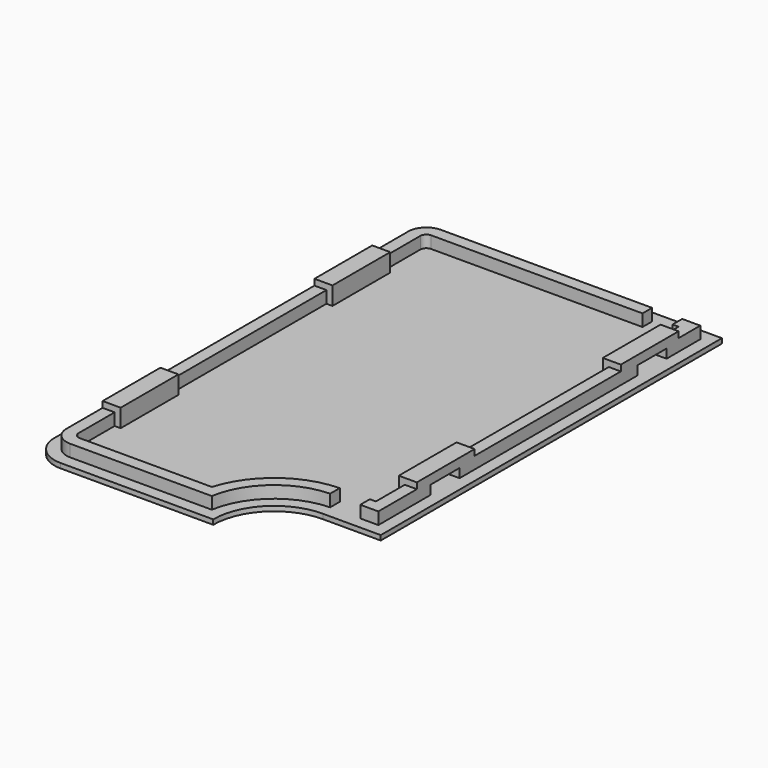
from build123d import *

# Parameters (mm, degrees)
F1_DEPTH  = 0.8
F2_R      = 5
F3_R      = 5
F5_DEPTH  = 3
F8_W      = 6
F8_H      = 1.5
F9_DEPTH  = 2
F11_DEPTH = 1.5
F12_DEPTH = 1.5
F6_W      = 6
F6_H      = 1.5
F13_DEPTH = 1
F14_W     = 2
F14_H     = 32
F14_H_2   = 30.375
F15_DEPTH = 2


# Not quite as in the source:
# - an extrude ends at something that could not be found from the text; its depth is read off the source's solid


with BuildPart() as f1:
    # F0 (on Top) → F1 (new body)
    with BuildSketch(Plane.XY):
        with BuildLine():
            Line((20.9010709455, 49.8366734011), (-29.2176790545, 49.8366734011))
            Line((-29.2176790545, 49.8366734011), (-29.2176790545, -31.1633265989))
            Line((-29.2176790545, -31.1633265989), (1.1573209455, -31.1633265989))
            ThreePointArc((1.1573209455, -31.1633265989), (4.122864786, -24.0038704394), (11.2823209455, -21.0383265989))
            Line((11.2823209455, -21.0383265989), (20.9010709455, -21.0383265989))
            Line((20.9010709455, -21.0383265989), (20.9010709455, 49.8366734011))
        make_face()
    extrude(amount=F1_DEPTH)

    # F2
    f2_edges = [f1.edges().sort_by_distance(p)[0] for p in [
        (-29.217679, 49.836673, 0.4),
    ]]
    fillet(f2_edges, radius=F2_R)

    # F3
    f3_edges = [f1.edges().sort_by_distance(p)[0] for p in [
        (-29.217679, -31.163327, 0.4),
    ]]
    fillet(f3_edges, radius=F3_R)

    # F4 (on face) → F5 (join)
    with BuildSketch(Plane.XY.offset(0.8)):
        with BuildLine():
            ThreePointArc((-24.2176790545, 47.8366734011), (-26.338999398, 46.9579937447), (-27.2176790545, 44.8366734011))
            Line((-27.2176790545, 44.8366734011), (-27.2176790545, -26.1633265989))
            ThreePointArc((-27.2176790545, -26.1633265989), (-26.338999398, -28.2846469425), (-24.2176790545, -29.1633265989))
            Line((-24.2176790545, -29.1633265989), (-0.6765930938, -29.1633265989))
            ThreePointArc((-0.6765930938, -29.1633265989), (3.4476025396, -21.9095267037), (11.2823209455, -19.0383265989))
            Line((11.2823209455, -19.0383265989), (18.9010709455, -19.0383265989))
            Line((18.9010709455, -19.0383265989), (18.9010709455, 47.8366734011))
            Line((18.9010709455, 47.8366734011), (-24.2176790545, 47.8366734011))
        make_face()
    extrude(amount=F5_DEPTH)

    # F8 (on face) → F9 (cut)
    with BuildSketch(Plane.YZ.offset(18.9010709455)):
        with Locations((-5.1633265989, 1.55)):
            Rectangle(F8_W, F8_H)
        with Locations((37.8366734011, 1.55)):
            Rectangle(F8_W, F8_H)
    extrude(amount=-F9_DEPTH, mode=Mode.SUBTRACT)

    # F10 (on face) → F11 (cut)
    with BuildSketch(Plane.XY.offset(3.8)):
        with BuildLine():
            Line((-24.2176790545, -18.6633265989), (-27.2176790545, -18.6633265989))
            Line((-27.2176790545, -18.6633265989), (-27.2176790545, -26.1633265989))
            ThreePointArc((-27.2176790545, -26.1633265989), (-26.338999398, -28.2846469425), (-24.2176790545, -29.1633265989))
            Line((-24.2176790545, -29.1633265989), (-0.6765930938, -29.1633265989))
            ThreePointArc((-0.6765930938, -29.1633265989), (3.4476025396, -21.9095267037), (11.2823209455, -19.0383265989))
            Line((11.2823209455, -19.0383265989), (18.9010709455, -19.0383265989))
            Line((18.9010709455, -19.0383265989), (18.9010709455, -11.0383265989))
            Line((18.9010709455, -11.0383265989), (15.9010709455, -11.0383265989))
            Line((15.9010709455, -11.0383265989), (15.9010709455, 0.9616734011))
            Line((15.9010709455, 0.9616734011), (18.9010709455, 0.9616734011))
            Line((18.9010709455, 0.9616734011), (18.9010709455, 31.3366734011))
            Line((18.9010709455, 31.3366734011), (15.9010709455, 31.3366734011))
            Line((15.9010709455, 31.3366734011), (15.9010709455, 43.3366734011))
            Line((15.9010709455, 43.3366734011), (18.9010709455, 43.3366734011))
            Line((18.9010709455, 43.3366734011), (18.9010709455, 47.8366734011))
            Line((18.9010709455, 47.8366734011), (-24.2176790545, 47.8366734011))
            ThreePointArc((-24.2176790545, 47.8366734011), (-26.338999398, 46.9579937447), (-27.2176790545, 44.8366734011))
            Line((-27.2176790545, 44.8366734011), (-27.2176790545, 37.3366734011))
            Line((-27.2176790545, 37.3366734011), (-24.2176790545, 37.3366734011))
            Line((-24.2176790545, 37.3366734011), (-24.2176790545, 25.3366734011))
            Line((-24.2176790545, 25.3366734011), (-27.2176790545, 25.3366734011))
            Line((-27.2176790545, 25.3366734011), (-27.2176790545, -6.6633265989))
            Line((-27.2176790545, -6.6633265989), (-24.2176790545, -6.6633265989))
            Line((-24.2176790545, -6.6633265989), (-24.2176790545, -18.6633265989))
        make_face()
    extrude(amount=-F11_DEPTH, mode=Mode.SUBTRACT)

    # F12 (cut, through all): a face of the model
    f12_faces = [f1.faces().sort_by_distance(p)[0] for p in [
        (-4.8878926555, 10.949585375, 2.3),
    ]]
    extrude(f12_faces, amount=-F12_DEPTH, mode=Mode.SUBTRACT)

    # F6 (on face) → F13 (cut)
    with BuildSketch(Plane(origin=(-27.2176790545, 0, 0), x_dir=(0, -1, 0), z_dir=(-1, 0, 0))):
        with Locations((-31.3366734011, 1.55)):
            Rectangle(F6_W, F6_H)
        with Locations((12.6633265989, 1.55)):
            Rectangle(F6_W, F6_H)
    extrude(amount=-F13_DEPTH, mode=Mode.SUBTRACT)

    # F14 (on face) → F15 (join)
    with BuildSketch(Plane.XY.offset(0.8)):
        with BuildLine():
            Line((-24.2176790545, -29.1633265989), (-0.6765930938, -29.1633265989))
            ThreePointArc((-0.6765930938, -29.1633265989), (3.3030681077, -22.0338606151), (10.9010709455, -19.04432196))
            Line((10.9010709455, -19.04432196), (10.9010709455, -17.0434727244))
            ThreePointArc((10.9010709455, -17.0434727244), (2.6741584042, -19.9644354635), (-2.2644729556, -27.1633265989))
            Line((-2.2644729556, -27.1633265989), (-24.2176790545, -27.1633265989))
            ThreePointArc((-24.2176790545, -27.1633265989), (-24.9247858357, -26.8704333801), (-25.2176790545, -26.1633265989))
            Line((-25.2176790545, -26.1633265989), (-25.2176790545, -18.6633265989))
            Line((-25.2176790545, -18.6633265989), (-27.2176790545, -18.6633265989))
            Line((-27.2176790545, -18.6633265989), (-27.2176790545, -26.1633265989))
            ThreePointArc((-27.2176790545, -26.1633265989), (-26.338999398, -28.2846469425), (-24.2176790545, -29.1633265989))
        make_face()
        Polygon((15.9010709455, -17.0383265989), (15.9010709455, -19.0383265989), (18.9010709455, -19.0383265989), (18.9010709455, -11.0383265989), (16.9010709455, -11.0383265989), (16.9010709455, -17.0383265989), align=None)
        Polygon((18.9010709455, 43.3366734011), (18.9010709455, 47.8366734011), (15.9010709455, 47.8366734011), (15.9010709455, 45.8366734011), (16.9010709455, 45.8366734011), (16.9010709455, 43.3366734011), align=None)
        with BuildLine():
            Line((10.9010709455, 47.8366734011), (-24.2176790545, 47.8366734011))
            ThreePointArc((-24.2176790545, 47.8366734011), (-26.338999398, 46.9579937447), (-27.2176790545, 44.8366734011))
            Line((-27.2176790545, 44.8366734011), (-27.2176790545, 37.3366734011))
            Line((-27.2176790545, 37.3366734011), (-25.2176790545, 37.3366734011))
            Line((-25.2176790545, 37.3366734011), (-25.2176790545, 44.8366734011))
            ThreePointArc((-25.2176790545, 44.8366734011), (-24.9247858357, 45.5437801823), (-24.2176790545, 45.8366734011))
            Line((-24.2176790545, 45.8366734011), (10.9010709455, 45.8366734011))
            Line((10.9010709455, 45.8366734011), (10.9010709455, 47.8366734011))
        make_face()
        with Locations((-26.2176790545, 9.3366734011)):
            Rectangle(F14_W, F14_H)
        with Locations((17.9010709455, 16.1491734011)):
            Rectangle(F14_W, F14_H_2)
    extrude(amount=F15_DEPTH)


solid = f1.part
